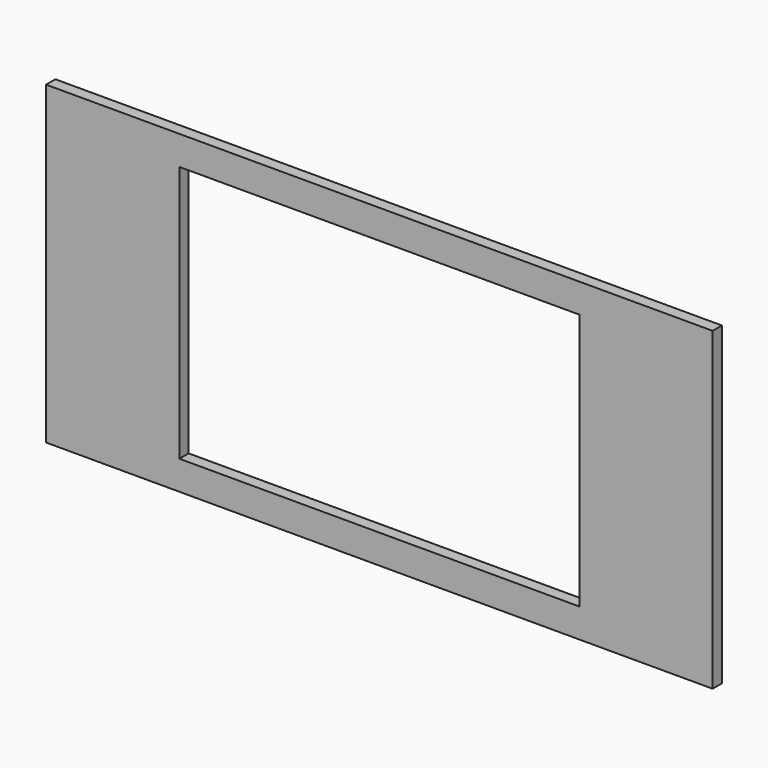
from build123d import *

# Parameters (mm, degrees)
F0_W     = 275
F0_H     = 130
F0_W_2   = 165
F0_H_2   = 106
F1_DEPTH = 4.8


# Not quite as in the source:
# - a feature names something its author has since deleted; it is built from what else it names


with BuildPart() as f1:
    # F0 (on Front) → F1 (new body)
    with BuildSketch(Plane.XZ):
        with Locations((-36.6599317901, 29.6020694077)):
            Rectangle(F0_W, F0_H)
        with Locations((-36.6599317901, 29.6020694077)):
            Rectangle(F0_W_2, F0_H_2, mode=Mode.SUBTRACT)
    extrude(amount=F1_DEPTH)


solid = f1.part
